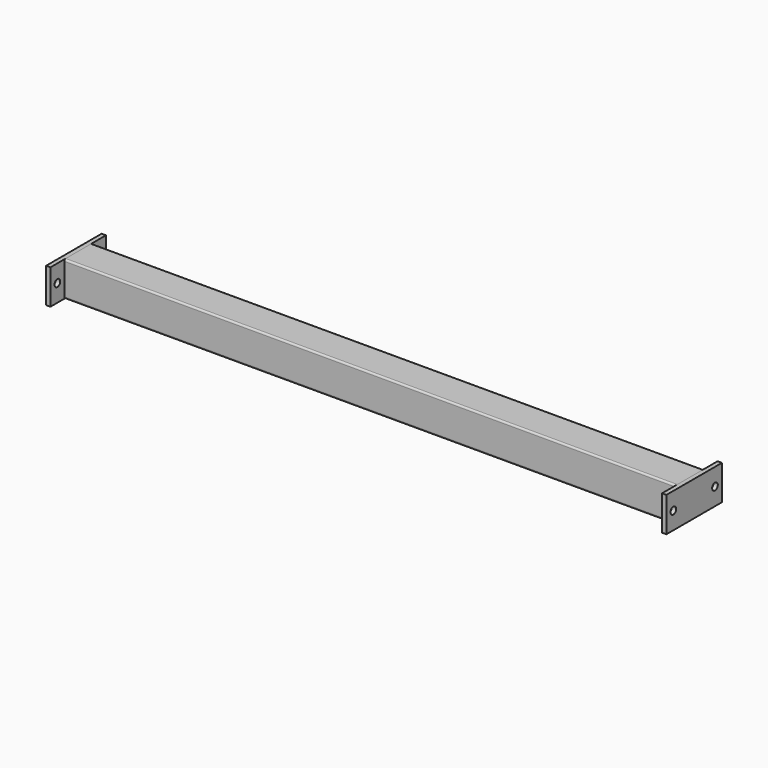
from build123d import *

# Parameters (mm, degrees)
F1_DEPTH = 447.675
F2_W     = 101.6
F2_H     = 50.8
F3_DEPTH = 6.35
F5_D     = 10.31875


# Not quite as in the source:
# - a length typed as a fraction of an inch, garbled in the dataset ("3 / 203.2 mm" for 3/8 in), is restored


with BuildPart() as f1:
    # F0 (on Right) → F1 (new body, symmetric)
    with BuildSketch(Plane.YZ):
        with BuildLine():
            ThreePointArc((25.4, 22.86), (24.6560512242, 24.6560512242), (22.86, 25.4))
            Line((22.86, 25.4), (-22.86, 25.4))
            ThreePointArc((-22.86, 25.4), (-24.6560512242, 24.6560512242), (-25.4, 22.86))
            Line((-25.4, 22.86), (-25.4, -22.86))
            ThreePointArc((-25.4, -22.86), (-24.6560512242, -24.6560512242), (-22.86, -25.4))
            Line((-22.86, -25.4), (22.86, -25.4))
            ThreePointArc((22.86, -25.4), (24.6560512242, -24.6560512242), (25.4, -22.86))
            Line((25.4, -22.86), (25.4, 22.86))
        make_face()
        with BuildLine():
            Line((-19.685, 22.225), (19.685, 22.225))
            ThreePointArc((19.685, 22.225), (21.4810512242, 21.4810512242), (22.225, 19.685))
            Line((22.225, 19.685), (22.225, -19.685))
            ThreePointArc((22.225, -19.685), (21.4810512242, -21.4810512242), (19.685, -22.225))
            Line((19.685, -22.225), (-19.685, -22.225))
            ThreePointArc((-19.685, -22.225), (-21.4810512242, -21.4810512242), (-22.225, -19.685))
            Line((-22.225, -19.685), (-22.225, 19.685))
            ThreePointArc((-22.225, 19.685), (-21.4810512242, 21.4810512242), (-19.685, 22.225))
        make_face(mode=Mode.SUBTRACT)
    extrude(amount=F1_DEPTH, both=True)


with BuildPart() as f3:
    # F2 (on face) → F3 (new body)
    with BuildSketch(Plane.YZ.offset(447.675)):
        Rectangle(F2_W, F2_H)
    extrude(amount=F3_DEPTH)

    # F5 (through all)
    with Locations(Plane.YZ.offset(454.025)):
        with Locations((-38.1, 0), (38.1, 0)):
            Hole(F5_D / 2)


with BuildPart() as f6_1:
    # F6: instance of F3
    add(f3.part.mirror(Plane.YZ))


solid = Compound([f1.part, f3.part, f6_1.part])
